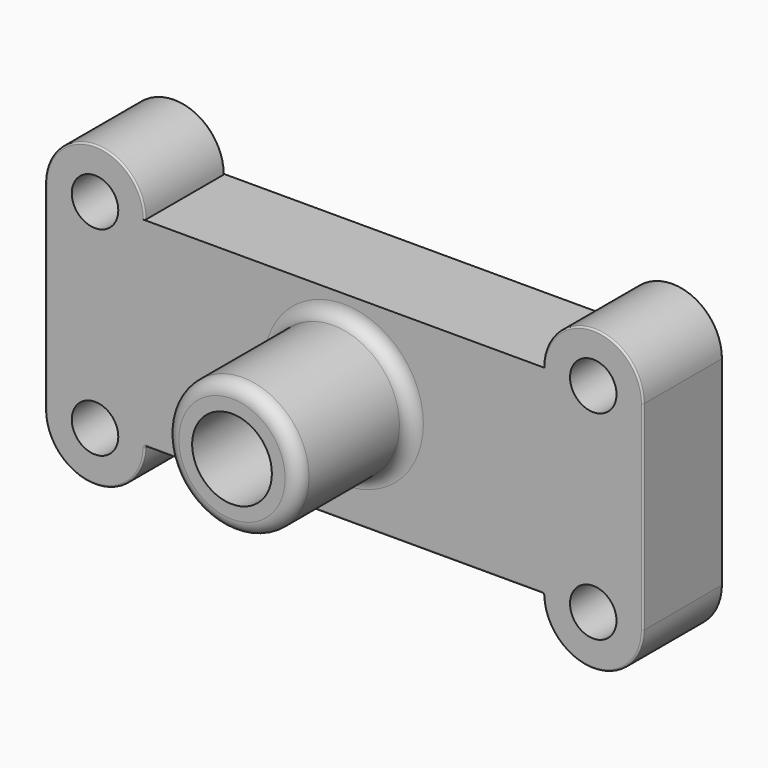
from build123d import *

# Parameters (mm, degrees)
F1_DEPTH = 15
F3_R     = 10
F4_DEPTH = 21
F5_R     = 6
F6_DEPTH = 36
F7_R     = 3.5
F8_DEPTH = 15.001
F9_R     = 2
F10_F1_R = 0.25
F10_F2_R = 0.25


with BuildPart() as f1:
    # F0 (on Front) → F1 (new body)
    with BuildSketch(Plane.XZ):
        with BuildLine():
            ThreePointArc((-15, 0), (-7.5, -7.5), (0, 0))
            Line((0, 0), (60, 0))
            ThreePointArc((60, 0), (67.5, -7.5), (75, 0))
            Line((75, 0), (75, 30))
            ThreePointArc((75, 30), (67.5, 37.5), (60, 30))
            Line((60, 30), (0, 30))
            ThreePointArc((0, 30), (-7.5, 37.5), (-15, 30))
            Line((-15, 30), (-15, 0))
        make_face()
    extrude(amount=F1_DEPTH)

    # F3 (on offset) → F4 (join, through all)
    with BuildSketch(Plane.XZ.offset(36)):
        with Locations((29.9208462238, 16.6226923466)):
            Circle(F3_R)
    extrude(amount=-F4_DEPTH)

    # F5 (on face) → F6 (cut, through all)
    with BuildSketch(Plane.XZ.offset(36)):
        with Locations((29.9208462238, 16.6226923466)):
            Circle(F5_R)
    extrude(amount=-F6_DEPTH, mode=Mode.SUBTRACT)

    # F7 (on face) → F8 (cut, through all)
    with BuildSketch(Plane.XZ.offset(15)):
        with Locations((-7.5, 30)):
            Circle(F7_R)
        with Locations((-7.5, 0)):
            Circle(F7_R)
        with Locations((67.5, 30)):
            Circle(F7_R)
        with Locations((67.5, 0)):
            Circle(F7_R)
    extrude(amount=-F8_DEPTH, mode=Mode.SUBTRACT)

    # F9
    f9_edges = [f1.edges().sort_by_distance(p)[0] for p in [
        (39.920846, -25.5, 16.622692),
        (19.920846, -36, 16.622692),
        (19.920846, -15, 16.622692),
    ]]
    fillet(f9_edges, radius=F9_R)

    # F10: fillet of radius 0.25 on 4 edges, made by hand

    # F10_f1
    f10_f1_edges = [f1.edges().sort_by_distance(p)[0] for p in [
        (0, -7.5, 0),
        (60, -7.5, 0),
    ]]
    fillet(f10_f1_edges, radius=F10_F1_R)

    # F10_f2
    f10_f2_edges = [f1.edges().sort_by_distance(p)[0] for p in [
        (30, 0, 0),
        (30, -15, 0),
        (0.0720646065, -15, -0.070394698),
        (59.9279353935, -15, -0.070394698),
        (0.0720646065, 0, -0.070394698),
        (59.9279353935, 0, -0.070394698),
    ]]
    fillet(f10_f2_edges, radius=F10_F2_R)


solid = f1.part
